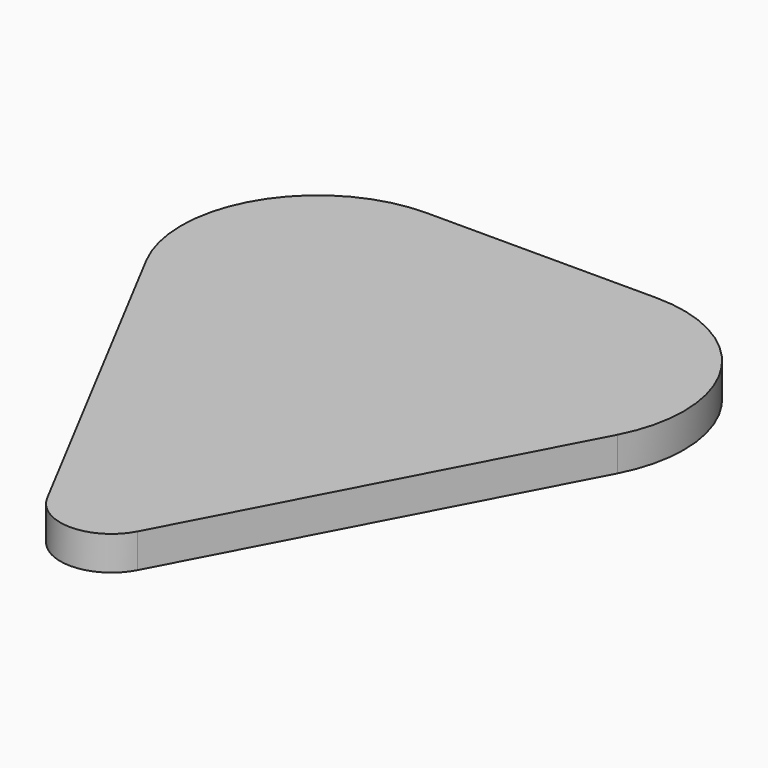
from build123d import *

# Parameters (mm, degrees)
F1_DEPTH = 1


# Not quite as in the source:
# - a feature of the source that left no trace in its solid (it failed there, or was rolled back) is left out


with BuildPart() as f1:
    # F0 (on Top) → F1 (new body, symmetric)
    with BuildSketch(Plane.XY):
        with BuildLine():
            Line((6.7490902932, 12.4546424842), (-6.7490902932, 12.4546424842))
            ThreePointArc((-6.7490902932, 12.4546424842), (-13.5977314614, 8.5893872344), (-13.8284360723, 0.7286710215))
            Line((-13.8284360723, 0.7286710215), (-2.6547546671, -20.5013236482))
            ThreePointArc((-2.6547546671, -20.5013236482), (0, -22.1040843497), (2.6547546671, -20.5013236482))
            Line((2.6547546671, -20.5013236482), (13.8284360723, 0.7286710215))
            ThreePointArc((13.8284360723, 0.7286710215), (13.5977314614, 8.5893872344), (6.7490902932, 12.4546424842))
        make_face()
    extrude(amount=F1_DEPTH, both=True)


solid = f1.part
